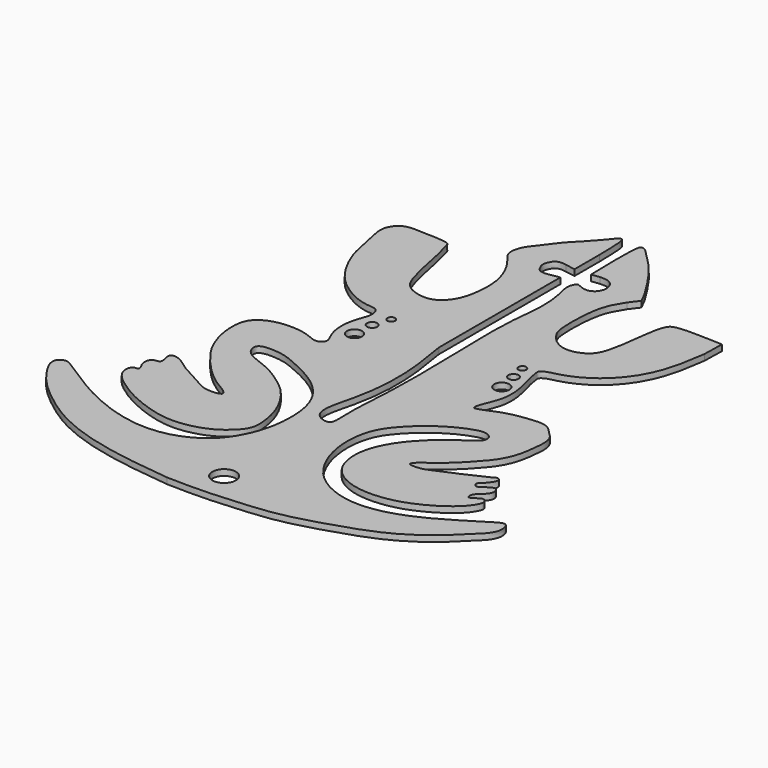
from build123d import *

# Parameters (mm, degrees)
F2_DEPTH = 5
F3_R     = 9.7959532295
F4_DEPTH = 25
F5_R     = 6.2931371703
F5_R_2   = 3.2460314562
F5_R_3   = 4.2194128036
F6_DEPTH = 5
F7_R     = 6.8726775006
F7_R_2   = 9.8092757214
F8_DEPTH = 3


# Not quite as in the source:
# - the dataset's text gives a spline's control points without its knots; the knots are read off the source's solid
# - a feature names something its author has since deleted; it is built from what else it names


with BuildPart() as f2:
    # F1 (on face) → F2 (new body)
    with BuildSketch(Plane.XY):
        with BuildLine():
            Line((-12.1370598, 172.6443334), (-4.0687244, 171.335065))
            Line((-4.0687244, 171.335065), (-4.0687244, 197.2649344))
            add(Edge.make_bspline(
                [(-27.7766018, -223.431481), (-42.9439324, -221.7688224), (-69.3382916, -218.8754068), (-104.974517, -210.7856592), (-135.4933028, -198.3873096), (-162.452812, -178.5535418), (-179.8535646, -161.5417394), (-191.2131812, -140.425805), (-181.778021, -135.1218786), (-173.8924132, -139.62634), (-153.4694162, -153.550874), (-119.580152, -173.0191358), (-72.4954862, -180.7496258), (-39.6882366, -165.642417), (-25.837769, -144.7113438), (-19.3576956, -127.0076962), (-17.2635418, -107.4295032), (-18.8454538, -88.2435116), (-26.8781784, -70.705472), (-42.3209466, -56.2935374), (-63.475997, -45.6827128), (-80.4761916, -39.0434068), (-99.5208576, -40.3158198), (-97.5535514, -49.9956074), (-92.4231324, -54.8033956), (-83.4681338, -58.390155), (-71.6334356, -62.8292368), (-59.1462876, -70.8907142), (-46.7704678, -80.4929048), (-37.6357896, -92.9368728), (-30.848808, -106.8625752), (-28.3535882, -119.6655468), (-27.4453604, -129.589276), (-29.756227, -137.0865432), (-35.896169, -144.1975272), (-45.6016106, -151.8789952), (-59.6664796, -157.0581568), (-80.0355778, -159.950404), (-105.824274, -152.7602736), (-128.5617952, -141.2028926), (-144.708753, -127.2310384), (-143.7711628, -118.6860212), (-142.4809444, -116.3416774), (-140.398119, -115.6690854), (-138.0413292, -115.9636492), (-137.775188, -113.152809), (-139.9324862, -110.298103), (-141.3748252, -105.8265092), (-140.1831842, -100.451412), (-136.499981, -99.191953), (-133.428994, -99.0864414), (-132.6657748, -96.2849484), (-133.6666364, -92.9647874), (-134.9575914, -86.240112), (-125.2704632, -87.3055404), (-116.17071, -95.981012), (-98.060002, -103.5003518), (-86.9984798, -112.3796838), (-71.7223356, -109.6558894), (-75.0191032, -105.7989248), (-77.344397, -103.9134066), (-84.6842858, -99.947349), (-96.0875904, -91.5853896), (-109.2976224, -77.4469114), (-120.505093, -61.9062008), (-126.283339, -45.6405234), (-128.1219942, -31.1927748), (-126.186565, -17.1450508), (-113.9238006, -8.45058), (-97.9116406, -6.5086992), (-83.2433438, -8.0086708), (-72.6547188, -14.1473682), (-65.1235934, -8.8223598), (-70.223507, -0.237998), (-72.656065, 8.7114126), (-72.7362528, 20.188682), (-69.6930534, 30.4376582), (-66.2154632, 39.1742168), (-69.2340246, 47.4719904), (-78.4831552, 47.5397576), (-88.8852172, 50.3521726), (-100.8126762, 57.0014608), (-113.1569746, 67.1551362), (-123.1774524, 81.988914), (-131.4553378, 100.9303798), (-134.008114, 120.7061086), (-139.545949, 138.3089182), (-128.7590516, 152.0287282), (-114.953288, 149.546945), (-103.3233392, 150.0379016), (-96.6186536, 149.2910654), (-90.647901, 148.5139778), (-89.41435, 141.6490182), (-86.7780586, 133.636639), (-83.7308714, 118.011448), (-80.5016424, 101.9233928), (-74.745088, 85.7471488), (-62.7137176, 79.5542224), (-48.2167946, 78.4393656), (-35.8062022, 91.8420566), (-32.91459, 108.5912738), (-32.6885554, 125.4421418), (-37.1278658, 140.3067806), (-44.1028074, 152.0629166), (-52.6540984, 161.0437216), (-51.1619246, 173.0820008), (-42.386123, 184.2285876), (-30.1284132, 200.7351586), (-19.6364352, 208.9383934), (-6.4808862, 227.2961672), (-4.5579538, 217.3012418), (-4.2870628, 209.3213492), (-4.1491408, 201.7053116), (-4.0687244, 197.2649344)],
                knots=[0, 0, 0, 0, 1.802021, 3.135895, 4.294727, 5.697075, 6.91816, 7.569791, 7.74768, 8.021429, 8.546614, 10.761629, 12.521493, 13.998287, 14.69652, 15.441662, 16.20507, 17.006787, 17.6881, 18.426817, 19.470308, 20.372975, 20.859775, 21.071529, 21.354642, 21.674742, 22.199469, 22.847847, 23.420238, 24.039388, 24.652596, 25.23341, 25.574003, 25.815846, 26.13634, 26.666086, 27.263892, 27.882214, 29.074706, 30.291451, 31.075061, 31.196031, 31.28728, 31.368628, 31.450643, 31.510292, 31.64163, 31.873519, 32.050626, 32.217636, 32.299733, 32.376274, 32.508123, 32.74966, 32.944966, 33.392441, 34.318903, 35.075143, 35.348713, 35.440593, 35.573277, 35.723139, 36.410065, 37.243667, 37.996607, 38.657942, 39.251937, 39.726153, 40.235083, 40.882048, 41.599416, 41.991372, 42.17153, 42.501901, 42.929668, 43.33886, 43.815016, 44.195122, 44.427894, 44.710818, 45.162458, 45.735867, 46.294007, 47.039374, 47.828514, 48.698131, 49.442813, 49.820919, 50.528531, 50.908453, 51.204472, 51.356697, 51.543141, 51.920858, 52.410129, 53.38516, 53.916214, 54.319474, 54.919717, 55.48325, 56.282491, 56.885471, 57.465171, 58.079609, 58.516734, 58.833919, 59.403097, 60.197628, 61.097718, 61.575093, 61.720475, 62.088314, 62.602639, 62.602639, 62.602639, 62.602639], degree=3))
            Line((-27.7766018, -223.431481), (-27.7764748, -223.4316842))
            add(Edge.make_bspline(
                [(136.5942912, 130.7330634), (134.7158342, 117.7473388), (131.0860726, 92.6546534), (109.6158844, 61.7602524), (86.8905806, 50.2379996), (73.36536, 47.5638368), (70.035928, 46.1924654), (67.278504, 44.0729878), (67.979925, 39.9304764), (68.6636676, 34.920555), (71.2338936, 25.9231892), (74.0970578, 14.748002), (74.0415588, 0.980821), (70.4443346, -8.647938), (67.5547544, -15.7001718), (66.4692346, -19.1075818), (66.4881576, -22.7258626), (70.320408, -21.7005408), (73.9749092, -20.6322422), (79.681832, -17.8995832), (86.7883202, -15.271496), (95.2360046, -13.201015), (104.706547, -11.9931688), (113.2135404, -10.9986572), (121.4861172, -12.9591054), (126.3829832, -18.5827162), (132.0438558, -23.4965748), (133.9628766, -31.9477644), (132.8568082, -40.8288236), (131.8326294, -50.5403358), (129.404872, -59.1310476), (124.7978708, -68.9421786), (115.7198346, -79.8662106), (103.926767, -92.096209), (93.6054008, -100.1682782), (86.961218, -104.9345628), (84.8076028, -106.958003), (82.5447676, -110.6020394), (93.5331378, -111.4323654), (102.9423646, -106.411649), (117.7368232, -100.9359424), (129.3340822, -94.52483), (136.2310458, -92.3470594), (140.9305792, -88.8064518), (143.9430192, -92.1330644), (141.4422622, -96.4649074), (138.8454678, -100.3514122), (133.2897766, -104.1512522), (137.4367584, -108.8507348), (142.4969972, -104.7131764), (148.8753182, -100.2815622), (152.5306576, -107.8972696), (146.9618854, -113.722658), (141.7570698, -117.6484058), (142.2106122, -124.336175), (147.8976214, -120.3519818), (152.1534422, -117.6472882), (155.8719514, -122.0046328), (152.4945388, -129.6355802), (144.3325282, -138.5899692), (130.2481012, -147.925409), (111.6803202, -156.3402512), (90.601927, -159.7436226), (69.5513976, -156.713936), (50.891821, -144.4060358), (44.9905374, -118.0277294), (57.5192652, -89.3146042), (78.11389, -70.2691254), (93.3718732, -59.8313764), (101.84765, -53.6060904), (100.284661, -46.9826594), (94.266766, -44.128563), (85.4493846, -46.2144618), (73.7099618, -51.0878328), (59.795664, -59.8932508), (47.0055956, -71.5245966), (34.4063066, -87.2153196), (30.2451008, -110.5835736), (35.1330768, -136.6508316), (50.438304, -162.2783902), (81.3077622, -177.6120654), (121.1732654, -173.4205066), (153.5451082, -155.1985212), (172.0513196, -143.1765996), (185.8317848, -135.025765), (190.3115066, -148.6768172), (175.1566728, -163.5612172), (156.1538152, -182.249953), (130.3357058, -197.2979036), (104.6655514, -206.4350456), (81.9149746, -213.551262), (57.479438, -219.6462206), (29.4467534, -222.0781944), (0.4016248, -224.0965546), (-19.3840862, -223.6297026), (-27.7764748, -223.4316842)],
                knots=[0, 0, 0, 0, 1.535148, 2.96641, 4.24803, 4.431746, 4.583926, 4.680176, 4.806754, 5.028953, 5.301828, 5.898185, 6.395491, 6.891904, 7.112044, 7.27483, 7.353428, 7.447161, 7.62871, 7.863296, 8.166905, 8.532315, 8.884042, 9.295487, 9.540963, 9.847306, 10.154769, 10.403481, 10.82816, 11.210681, 11.555165, 11.877281, 12.483453, 13.220061, 13.87865, 14.039327, 14.170389, 14.249126, 14.458283, 14.997072, 15.780622, 16.216936, 16.543879, 16.691134, 16.790875, 16.96249, 17.191057, 17.426886, 17.531666, 17.773319, 18.070303, 18.222833, 18.5719, 18.885447, 18.980312, 19.200437, 19.411041, 19.524196, 19.766268, 20.272911, 20.998847, 21.721386, 22.676898, 23.474372, 24.19237, 25.171857, 26.36393, 27.75309, 28.365686, 28.666119, 28.839884, 29.06278, 29.372446, 29.878107, 30.570731, 31.299421, 31.918778, 32.910411, 33.97722, 35.009659, 36.324801, 37.785722, 39.611746, 40.436885, 40.791288, 41.01349, 41.796249, 43.01555, 44.294075, 45.241835, 46.238982, 47.108257, 48.209548, 49.554848, 50.545806, 50.545806, 50.545806, 50.545806], degree=3))
            Line((136.5942912, 130.7330634), (136.9948238, 148.5141556))
            Line((136.9948238, 148.5141556), (118.0072316, 149.193504))
            add(Edge.make_bspline(
                [(51.9556238, 156.162375), (49.6509294, 152.4989076), (44.7408808, 144.6940718), (41.5128964, 129.5920192), (40.8840178, 115.055015), (41.0337762, 102.9993114), (42.360977, 94.8553602), (46.5868004, 88.1687086), (52.6237454, 82.1952128), (61.8679738, 79.0324302), (71.3963012, 80.5552618), (81.2663856, 86.3031548), (86.0913696, 101.4344428), (87.9530372, 117.3879288), (89.8982962, 132.4399434), (91.7143454, 141.3805656), (94.5295798, 147.3280264), (100.4390422, 148.824315), (108.0464946, 149.4339912), (114.3100584, 149.2827596), (118.0072316, 149.193504)],
                knots=[0, 0, 0, 0, 0.507801, 1.081846, 1.794622, 2.225848, 2.509031, 2.751823, 3.147595, 3.490879, 3.860873, 4.26059, 4.767083, 5.637274, 6.192749, 6.542565, 6.734152, 6.915163, 7.216783, 7.6513, 7.6513, 7.6513, 7.6513], degree=3))
            Line((51.9556238, 156.162375), (57.7270372, 163.8106198))
            Line((57.7270372, 163.8106198), (53.1311612, 172.8192124))
            add(Edge.make_bspline(
                [(8.5070442, 196.4388502), (8.4782914, 200.638537), (8.428228, 207.9533052), (8.7244174, 215.842596), (10.2165658, 226.2216964), (27.2943828, 208.9815988), (38.2146048, 196.8283338), (48.104044, 180.9106618), (53.1311612, 172.8192124)],
                knots=[0, 0, 0, 0, 0.487171, 0.84853, 1.009311, 1.51751, 2.549012, 3.615474, 3.615474, 3.615474, 3.615474], degree=3))
            Line((8.5070442, 196.4388502), (9.0487246, 172.222287))
            Line((9.0487246, 172.222287), (15.6550868, 173.0011272))
            add(Edge.make_bspline(
                [(-4.0684704, 30.0780958), (0.6444234, 2.3602188), (7.0374256, -35.2388932), (-12.9332228, -93.8166526), (8.433308, -98.5416876), (6.9033898, -73.9753156), (10.4568752, -38.2939798), (10.1170994, 24.6197628), (7.4708004, 86.6945434), (14.7446238, 126.7812044), (6.0599574, 150.5767626), (10.9620812, 156.0520628), (12.8937766, 155.3455364), (15.996412, 153.8545056), (21.4429594, 152.488011), (27.5881592, 156.0329112), (29.7631612, 162.4870512), (28.161488, 168.95953), (22.568281, 173.2302606), (18.1009036, 173.082204), (15.6550868, 173.0011272)],
                knots=[0, 0, 0, 0, 3.657987, 4.962035, 5.231976, 5.650516, 7.118406, 10.203105, 12.671445, 14.451119, 15.156835, 15.191561, 15.259473, 15.361827, 15.624539, 15.869057, 16.123989, 16.376066, 16.608867, 16.890525, 16.890525, 16.890525, 16.890525], degree=3))
            Line((-4.0684704, 30.0780958), (-4.0684704, 156.5139364))
            Line((-4.0684704, 156.5139364), (-12.1370598, 155.204668))
            add(Edge.make_bspline(
                [(-12.1370598, 172.6443334), (-13.8639296, 172.947711), (-16.7183054, 173.4491832), (-20.9770726, 172.2433436), (-22.9520496, 168.9792404), (-24.4239796, 165.7488684), (-24.4239796, 162.100133), (-22.9520496, 158.869761), (-20.977098, 155.6056324), (-16.7183054, 154.3997928), (-13.8639296, 154.901265), (-12.1370598, 155.204668)],
                knots=[0, 0, 0, 0, 0.20618, 0.340799, 0.489945, 0.634795, 0.759592, 0.904443, 1.05359, 1.188209, 1.394389, 1.394389, 1.394389, 1.394389], degree=3))
        make_face()
    extrude(amount=F2_DEPTH)

    # F3 (on face) → F4 (cut)
    with BuildSketch(Plane.XY.offset(5)):
        with Locations((0, -198.7284123898)):
            Circle(F3_R)
    extrude(amount=-F4_DEPTH, mode=Mode.SUBTRACT)

    # F5 (on face) → F6 (cut)
    with BuildSketch(Plane.XY):
        with Locations((62.6488402486, 12.166804634)):
            Circle(F5_R)
        with Locations((-59.0279139578, 10.8311446384)):
            Circle(F5_R)
        with Locations((-53.0001819134, 41.5725894272)):
            Circle(F5_R_2)
        with Locations((59.7815550864, 27.9368981719)):
            Circle(F5_R_3)
        with Locations((-57.8223690391, 27.7087986469)):
            Circle(F5_R_3)
        with Locations((56.7045807838, 40.9698113799)):
            Circle(F5_R_2)
    extrude(amount=F6_DEPTH, mode=Mode.SUBTRACT)

    # F7 (on face) → F8 (join)
    with BuildSketch(Plane.XY):
        with Locations((-68.3831125498, -196.0495710373)):
            Circle(F7_R)
        with Locations((-39.2295047641, -198.1505304575)):
            Circle(F7_R_2)
        with BuildLine():
            Line((-93.2197421789, -196.9460760807), (-93.2197421789, -186.0294128204))
            ThreePointArc((-93.2197421789, -186.0294128204), (-98.6780738091, -191.4877444506), (-93.2197421789, -196.9460760807))
        make_face()
        with Locations((37.2056253254, -198.0363726616)):
            Circle(F7_R_2)
    extrude(amount=-F8_DEPTH)


solid = f2.part
